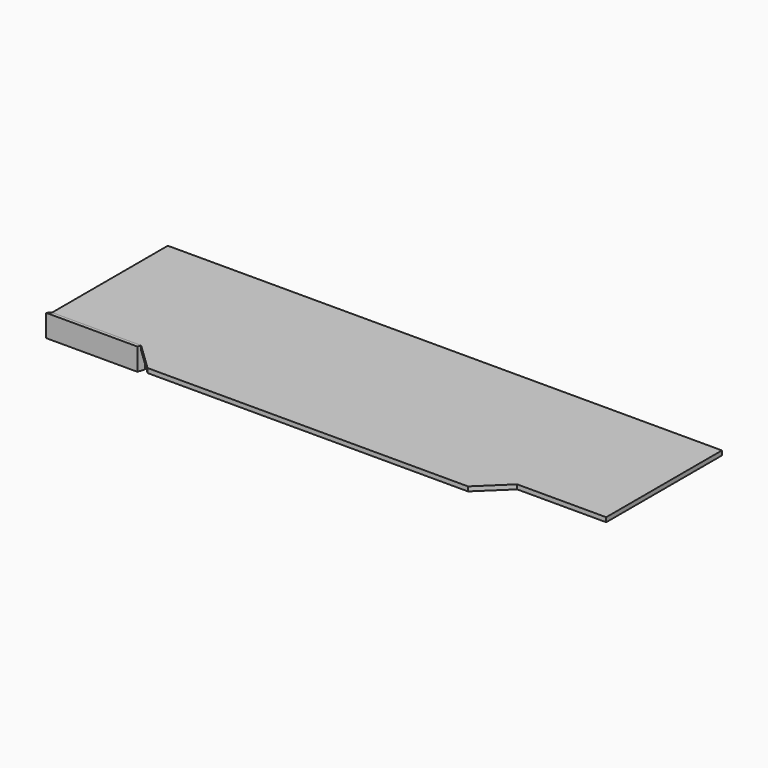
from build123d import *

# Parameters (mm, degrees)
F1_DEPTH      = 12.7
F3_DEPTH      = 50.8
F3_DEPTH_BACK = 12.7
F5_DEPTH      = 50.8


with BuildPart() as f1:
    # F0 (on Top) → F1 (new body)
    with BuildSketch(Plane.XY):
        Polygon((790.575, 0), (-790.575, 0), (-790.575, -412.75), (-536.575, -412.75), (-457.2, -488.95), (457.2, -488.95), (536.575, -412.75), (790.575, -412.75), align=None)
    extrude(amount=F1_DEPTH)


with BuildPart() as f3:
    # F2 (on face) → F3 (new body, two sides)
    with BuildSketch(Plane(origin=(0, 0, 0), x_dir=(1, 0, 0), z_dir=(0, 0, -1))) as f3_sk:
        Polygon((-800.1, 422.275), (-790.575, 412.75), (-536.575, 412.75), (-539.6698601066, 422.275), align=None)
    extrude(amount=F3_DEPTH)
    extrude(f3_sk.sketch, amount=-F3_DEPTH_BACK)

    # F4 (on face) → F5 (join)
    with BuildSketch(Plane(origin=(0, 0, -50.8), x_dir=(1, 0, 0), z_dir=(0, 0, -1))):
        Polygon((-536.575, 412.75), (-790.575, 412.75), (-781.05, 403.225), (-533.4801398934, 403.225), align=None)
    extrude(amount=-F5_DEPTH)


solid = Compound([f1.part, f3.part])
